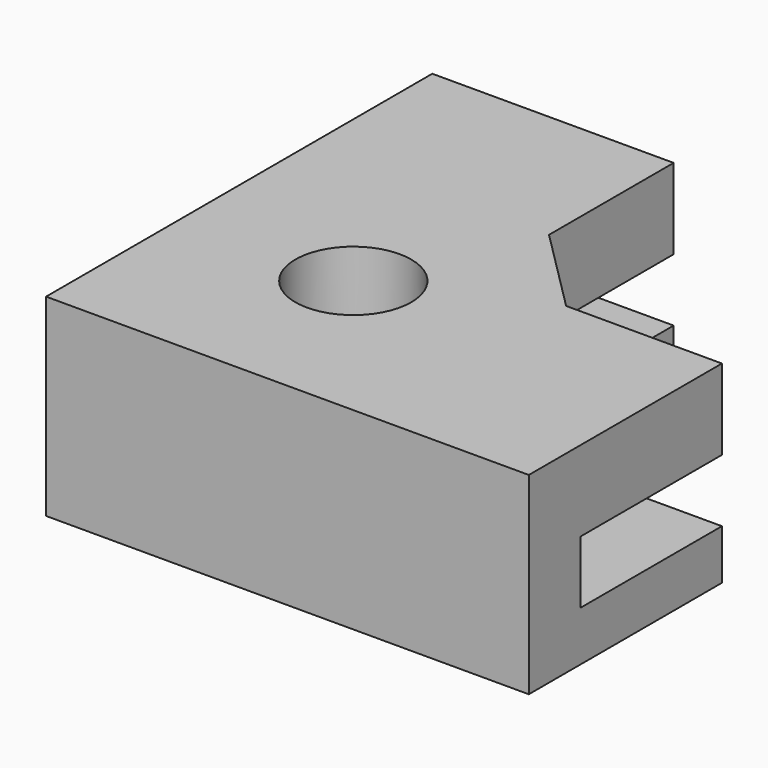
from build123d import *

# Parameters (mm, degrees)
F0_W     = 4
F0_H     = 15
F0_W_2   = 11
F0_H_2   = 11
F0_R     = 3.6
F0_H_3   = 4
F0_R_2   = 1.6
F1_DEPTH = 12
F2_START = 3.1
F2_DEPTH = 3.9
F3_START = 5
F3_DEPTH = 5
F4_START = 3.3
F4_DEPTH = 19.2


# Not quite as in the source:
# - a feature names something its author has since deleted; it is built from what else it names


with BuildPart() as f1:
    # F0 (on Top) → F1 (new body)
    with BuildSketch(Plane.XY):
        with Locations((-13, 7.5)):
            Rectangle(F0_W, F0_H)
        Polygon((-11, 0), (0, 0), (0, 5.31885653), (0, 15), (-7, 15), (-11, 15), align=None)
        Polygon((0, -11), (15, -11), (15, -7), (15, 0), (5.31885653, 0), (0, 0), align=None)
        Polygon((2.9605122421, -15), (15, -15), (15, -11), (0, -11), (0, -15), align=None)
        with Locations((-5.5, -5.5)):
            Rectangle(F0_W_2, F0_H_2)
        with Locations((-4.3933982822, -4.3933982822)):
            Circle(F0_R, mode=Mode.SUBTRACT)
        Polygon((0, 5.31885653), (0, 0), (5.31885653, 0), align=None)
        with Locations((-13, -13)):
            Rectangle(F0_W, F0_H_3)
        Polygon((-15, -11), (-11, -11), (-11, 0), (-15, 0), (-15, -7), align=None)
        with Locations((-5.5, -13)):
            Rectangle(F0_W_2, F0_H_3)
        with Locations((-4.3933982822, -4.3933982822)):
            Circle(F0_R)
        with Locations((-4.3933982822, -4.3933982822)):
            Circle(F0_R_2, mode=Mode.SUBTRACT)
    extrude(amount=F1_DEPTH)

    # F0 (on Top) → F2 (cut)
    with BuildSketch(Plane.XY.offset(F2_START)):
        Polygon((0, -11), (15, -11), (15, -7), (15, 0), (5.31885653, 0), (0, 0), align=None)
        with Locations((-5.5, -5.5)):
            Rectangle(F0_W_2, F0_H_2)
        with Locations((-4.3933982822, -4.3933982822)):
            Circle(F0_R, mode=Mode.SUBTRACT)
        Polygon((-11, 0), (0, 0), (0, 5.31885653), (0, 15), (-7, 15), (-11, 15), align=None)
        Polygon((0, 5.31885653), (0, 0), (5.31885653, 0), align=None)
    extrude(amount=F2_DEPTH, mode=Mode.SUBTRACT)

    # F0 (on Top) → F3 (cut)
    with BuildSketch(Plane.XY.offset(F3_START)):
        Polygon((0, 5.31885653), (0, 0), (5.31885653, 0), align=None)
    extrude(amount=F3_DEPTH, mode=Mode.SUBTRACT)

    # F0 (on Top) → F4 (cut)
    with BuildSketch(Plane.XY.offset(F4_START)):
        with Locations((-4.3933982822, -4.3933982822)):
            Circle(F0_R)
        with Locations((-4.3933982822, -4.3933982822)):
            Circle(F0_R_2, mode=Mode.SUBTRACT)
    extrude(amount=F4_DEPTH, mode=Mode.SUBTRACT)


solid = f1.part
